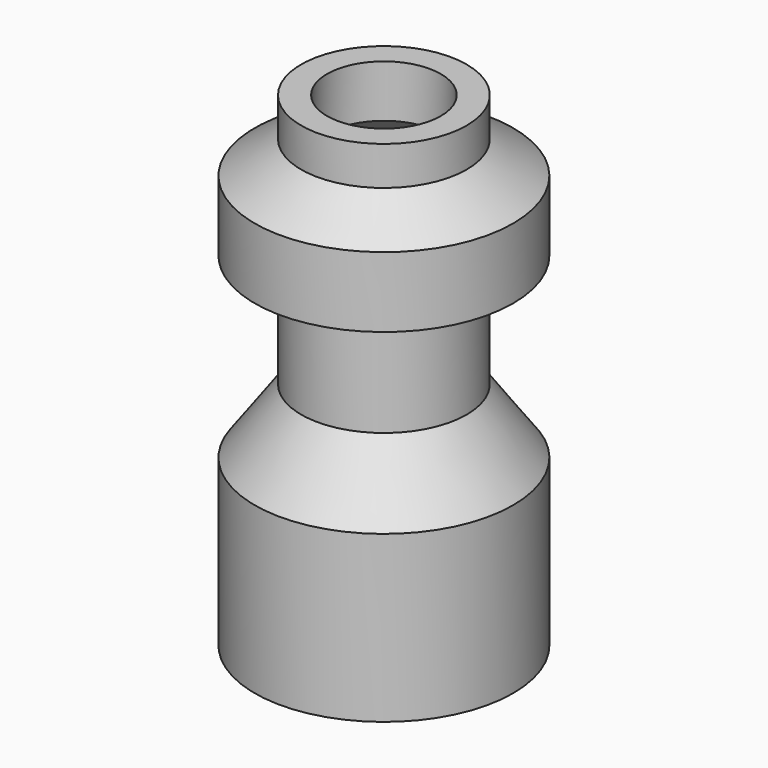
from build123d import *

# Parameters (mm, degrees)
F2_T = -8


with BuildPart() as f1:
    # F0 (on Front) → F1 (revolve)
    with BuildSketch(Plane.XZ):
        Polygon((0, 150), (0, 0), (40, 0), (40, 51.2300857674), (25.6093478629, 71.2300857674), (25.6093478629, 101.2300857674), (40, 106.2300857674), (40, 128), (25.6093478629, 138), (25.6093478629, 150), align=None)
    revolve(axis=Axis((0, 0, 75), (0, 0, -1)))

    # F2
    f2_openings = [f1.faces().sort_by_distance(p)[0] for p in [
        (0, 0, 150),
    ]]
    offset(amount=F2_T, openings=f2_openings, kind=Kind.INTERSECTION)


solid = f1.part
